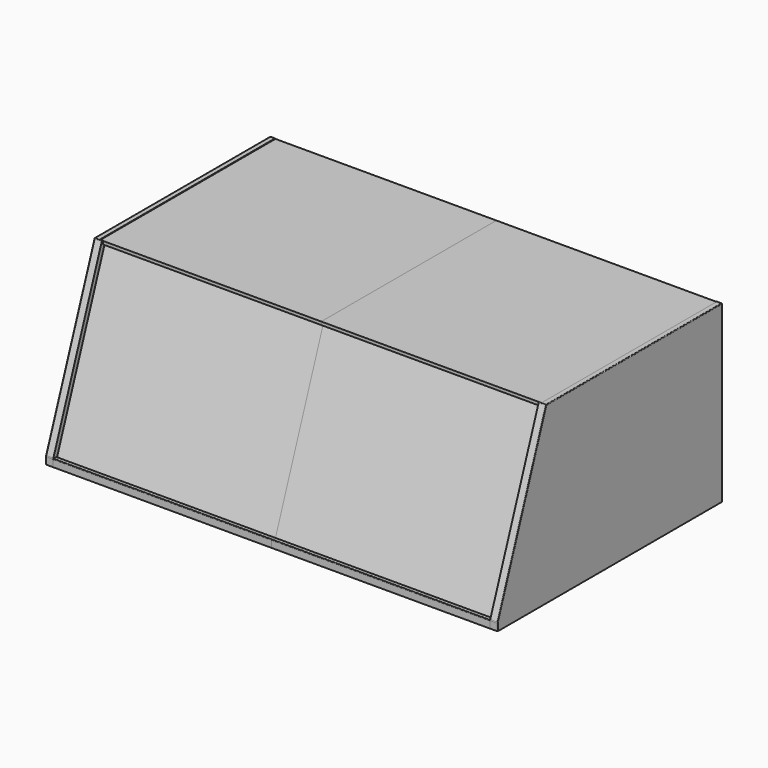
from build123d import *

# Parameters (mm, degrees)
F2_W         = 350
F2_H         = 450
F3_DEPTH     = 12
F5_DEPTH     = 12
F6_DEPTH     = 4
F8_DEPTH     = 354
F9_DEPTH     = 354
F10_W        = 7.1407400337
F10_H        = 5
F11_DEPTH    = 350.001
F12_R        = 1
F12_2_R      = 1
F13_T1_DEPTH = 14.2040872589
F13_T4_ANGLE = 20


# Not quite as in the source:
# - a fillet or chamfer that OpenCascade refuses, or shapes differently, is made with other operations: its cross-section is extruded or revolved along the edge and cut away or added


with BuildPart() as f3:
    # F2 (on Top) → F3 (new body)
    with BuildSketch(Plane.XY):
        with Locations((-175, 225)):
            Rectangle(F2_W, F2_H)
    extrude(amount=F3_DEPTH)

    # F10 (on face) → F11 (cut, through all)
    with BuildSketch(Plane(origin=(-350, 0, 0), x_dir=(0, -1, 0), z_dir=(-1, 0, 0))):
        with Locations((-9.7318521391, 9.5)):
            Rectangle(F10_W, F10_H)
    extrude(amount=-F11_DEPTH, mode=Mode.SUBTRACT)

    # F12
    f12_edges = [f3.edges().sort_by_distance(p)[0] for p in [
        (-175, 0, 12),
        (-175, 450, 12),
    ]]
    fillet(f12_edges, radius=F12_R)


with BuildPart() as f5:
    # F4 (on face) → F5 (new body)
    with BuildSketch(Plane(origin=(-350, 0, 0), x_dir=(0, -1, 0), z_dir=(-1, 0, 0))):
        Polygon((-450, 12), (-450, 0), (0, 0), (0, 12), (-7.9813332936, 12), (-6.1614821222, 7), (-11.4823709846, 7), (-13.3022221559, 12), align=None)
        Polygon((-7.9813332936, 12), (-13.3022221559, 12), (-11.4823709846, 7), (-6.1614821222, 7), align=None)
        Polygon((-7.9813332936, 12), (0, 12), (-97.5440227833, 280), (-99.3415346713, 280), (-99.3415346713, 274), (-103.3415346713, 274), align=None)
        Polygon((-108.6624235337, 274), (-13.3022221559, 12), (-7.9813332936, 12), (-103.3415346713, 274), align=None)
        Polygon((-450, 274), (-450, 12), (-13.3022221559, 12), (-108.6624235337, 274), align=None)
        Polygon((-99.3415346713, 274), (-99.3415346713, 280), (-105.5253560769, 280), (-103.3415346713, 274), align=None)
        Polygon((-110.8462449393, 280), (-108.6624235337, 274), (-103.3415346713, 274), (-105.5253560769, 280), align=None)
        Polygon((-450, 280), (-450, 274), (-108.6624235337, 274), (-110.8462449393, 280), align=None)
    extrude(amount=F5_DEPTH)

    # F4 (on face) → F6 (cut)
    with BuildSketch(Plane(origin=(-350, 0, 0), x_dir=(0, -1, 0), z_dir=(-1, 0, 0))):
        Polygon((-7.9813332936, 12), (-13.3022221559, 12), (-11.4823709846, 7), (-6.1614821222, 7), align=None)
        Polygon((-108.6624235337, 274), (-13.3022221559, 12), (-7.9813332936, 12), (-103.3415346713, 274), align=None)
        Polygon((-99.3415346713, 274), (-99.3415346713, 280), (-105.5253560769, 280), (-103.3415346713, 274), align=None)
        Polygon((-110.8462449393, 280), (-108.6624235337, 274), (-103.3415346713, 274), (-105.5253560769, 280), align=None)
        Polygon((-450, 280), (-450, 274), (-108.6624235337, 274), (-110.8462449393, 280), align=None)
    extrude(amount=F6_DEPTH, mode=Mode.SUBTRACT)

    # F12#2
    f12_2_edges = [f5.edges().sort_by_distance(p)[0] for p in [
        (-362, 48.772011, 146),
        (-362, 273.772011, 280),
        (-356, 97.544023, 280),
        (-362, 450, 140),
        (-362, 0, 6),
        (-358, 450, 280),
    ]]
    fillet(f12_2_edges, radius=F12_2_R)

    # F13: fillet of radius 5 on 1 edges, made by hand

    # F13_s2 → F13_t1 (cut)
    with BuildSketch(Plane.YZ.offset(-362)):
        with BuildLine():
            ThreePointArc((0, 11.1183650965), (0.0759612349, 11.9866059848), (0.3015368961, 12.8284658131))
            Line((0.3015368961, 12.8284658131), (0, 12))
            Line((0, 12), (0, 11.1183650965))
        make_face()
    extrude(amount=F13_T1_DEPTH, mode=Mode.SUBTRACT)

    # F13_s3 → F13_t4 (revolve, cut)
    with BuildSketch(Plane.XY.offset(11.1183650965)):
        with BuildLine():
            ThreePointArc((-362, 1), (-361.7071067812, 0.2928932188), (-361, 0))
            Line((-361, 0), (-362, 0))
            Line((-362, 0), (-362, 1))
        make_face()
    revolve(axis=Axis((-362, 5, 11.1183650965), (-1, 0, 0)), revolution_arc=F13_T4_ANGLE, mode=Mode.SUBTRACT)


with BuildPart() as f8:
    # F7 (on face) → F8 (new body)
    with BuildSketch(Plane.YZ.offset(-354)):
        Polygon((103.3415346713, 274), (6.7839078807, 8.7101007166), (11.4823709846, 7), (108.6624235337, 274), align=None)
    extrude(amount=F8_DEPTH)


with BuildPart() as f9:
    # F7 (on face) → F9 (new body)
    with BuildSketch(Plane.YZ.offset(-354)):
        Polygon((99.3415346713, 274), (103.3415346713, 274), (108.6624235337, 274), (450, 274), (450, 279), (99.3415346713, 279), align=None)
    extrude(amount=F9_DEPTH)


with BuildPart() as f14_1:
    # F14: instance of F5
    add(f5.part.mirror(Plane(origin=(0, 226.4328970627, 5.9762405928), x_dir=(0, 1, 0), z_dir=(1, 0, 0))))


with BuildPart() as f14_2:
    # F14: instance of F9
    add(f9.part.mirror(Plane(origin=(0, 226.4328970627, 5.9762405928), x_dir=(0, 1, 0), z_dir=(1, 0, 0))))


with BuildPart() as f14_3:
    # F14: instance of F3
    add(f3.part.mirror(Plane(origin=(0, 226.4328970627, 5.9762405928), x_dir=(0, 1, 0), z_dir=(1, 0, 0))))


with BuildPart() as f14_4:
    # F14: instance of F8
    add(f8.part.mirror(Plane(origin=(0, 226.4328970627, 5.9762405928), x_dir=(0, 1, 0), z_dir=(1, 0, 0))))


solid = Compound([f3.part, f5.part, f8.part, f9.part, f14_1.part, f14_2.part, f14_3.part, f14_4.part])
